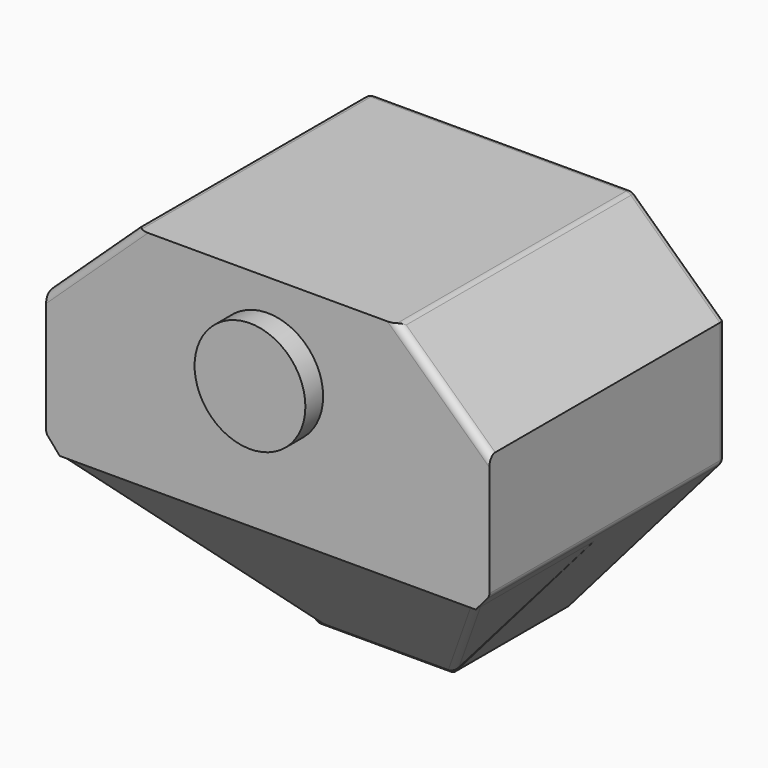
from build123d import *

# Parameters (mm, degrees)
F0_W          = 92.273324728
F0_H          = 57.6515942812
F0_W_2        = 42.1701818705
F0_H_2        = 26.3371020555
F0_H_3        = 119.797244668
F0_H_4        = 35.8085483313
F1_DEPTH      = 100
F1_DEPTH_BACK = 100
F3_DEPTH      = 100
F5_DEPTH      = 150
F5_DEPTH_BACK = 150
F7_DEPTH      = 100
F8_R          = 5
F9_T1_DEPTH   = 199.6642420397
F9_T3_DEPTH   = 100.7064549822
F9_T5_DEPTH   = 109.4378575727
F9_T7_DEPTH   = 199.9314988793
F9_T9_DEPTH   = 109.4378575727
F9_T11_DEPTH  = 200.4273166446
F9_T16_DEPTH  = 5.1
F9_T22_DEPTH  = 5.1
F9_T28_DEPTH  = 5.1
F9_T34_DEPTH  = 5.1
F9_T40_DEPTH  = 5.1
F9_T46_DEPTH  = 5.1
F9_T52_DEPTH  = 5.1
F9_T58_DEPTH  = 190.7815844726
F9_T64_DEPTH  = 191.1757464634
F10_R         = 37.5
F11_DEPTH     = 15
F12_W         = 12.8494501114
F12_H         = 17.9891586304
F13_DEPTH     = 50


# Not quite as in the source:
# - a fillet or chamfer that OpenCascade refuses, or shapes differently, is made with other operations: its cross-section is extruded or revolved along the edge and cut away or added


with BuildPart() as f1:
    # F0 (on Front) → F1 (new body, two sides)
    with BuildSketch(Plane.XZ) as f1_sk:
        with Locations((0, 13.1685510278)):
            Rectangle(F0_W, F0_H)
        with Locations((-67.2217532992, 13.1685510278)):
            Rectangle(F0_W_2, F0_H)
        Polygon((-150, 41.9943481684), (-150, -41.9943481684), (-46.136662364, -41.9943481684), (-46.136662364, -15.6572461128), (-88.3068442345, -15.6572461128), (-88.3068442345, 41.9943481684), align=None)
        with Locations((0, -28.8257971406)):
            Rectangle(F0_W, F0_H_2)
        Polygon((46.136662364, -15.6572461128), (46.136662364, -41.9943481684), (150, -41.9943481684), (150, 41.9943481684), (88.3068442345, 41.9943481684), (88.3068442345, -15.6572461128), align=None)
        with Locations((67.2217532992, 13.1685510278)):
            Rectangle(F0_W_2, F0_H)
        Polygon((-46.136662364, -41.9943481684), (-150, -41.9943481684), (-46.136662364, -161.7915928364), align=None)
        with Locations((0, -101.8929705024)):
            Rectangle(F0_W, F0_H_3)
        Polygon((150, -41.9943481684), (46.136662364, -41.9943481684), (46.136662364, -161.7915928364), align=None)
        Polygon((-88.3068442345, 99.6459424496), (-88.3068442345, 41.9943481684), (-46.136662364, 41.9943481684), (-46.136662364, 77.8028964996), (46.136662364, 77.8028964996), (46.136662364, 41.9943481684), (88.3068442345, 41.9943481684), (88.3068442345, 99.6459424496), align=None)
        with Locations((0, 59.898622334)):
            Rectangle(F0_W, F0_H_4)
        Polygon((-88.3068442345, 99.6459424496), (-150, 41.9943481684), (-88.3068442345, 41.9943481684), align=None)
        Polygon((150, 41.9943481684), (88.3068442345, 99.6459424496), (88.3068442345, 41.9943481684), align=None)
    extrude(amount=F1_DEPTH)
    extrude(f1_sk.sketch, amount=-F1_DEPTH_BACK)

    # F2 (on face) → F3 (cut)
    with BuildSketch(Plane.XZ.offset(100)):
        Polygon((140.7758174747, -52.633633175), (-140.7758174747, -52.633633175), (-46.136662364, -161.7915928364), (46.136662364, -161.7915928364), align=None)
    extrude(amount=-F3_DEPTH, mode=Mode.SUBTRACT)

    # F4 (on Right) → F5 (join, two sides)
    with BuildSketch(Plane.YZ) as f5_sk:
        Polygon((-99.6227860451, -52.5650829077), (0, -161.33877635), (0, -52.5650829077), align=None)
    extrude(amount=F5_DEPTH)
    extrude(f5_sk.sketch, amount=-F5_DEPTH_BACK)

    # F6 (on face) → F7 (cut)
    with BuildSketch(Plane.XZ.offset(100)):
        Polygon((-140.7758174747, -52.633633175), (-150, -41.9943481684), (-150.5579352379, -161.6920530796), (-44.7144806385, -161.6920530796), (-140.6417366282, -52.633633175), align=None)
        Polygon((140.7758174747, -52.633633175), (140.7202282019, -52.633633175), (45.5975532532, -161.6920530796), (150, -161.6920530796), (150, -41.9943481684), align=None)
    extrude(amount=-F7_DEPTH, mode=Mode.SUBTRACT)

    # F8
    f8_edges = [f1.edges().sort_by_distance(p)[0] for p in [
        (0, 100, 99.645942),
        (119.153422, 100, 70.820145),
        (-150, 100, 0),
        (-98.068331, 100, -101.892971),
        (0, 100, -161.791593),
        (98.068331, 100, -101.892971),
        (150, 100, 0),
        (-119.153422, 100, 70.820145),
    ]]
    fillet(f8_edges, radius=F8_R)

    # F9: fillet of radius 5 on 11 edges, made by hand

    # F9_s2 → F9_t1 (cut)
    with BuildSketch(Plane.XZ.offset(-95)):
        with BuildLine():
            ThreePointArc((148.7778357345, -43.4040073885), (149.6845052392, -41.8766246542), (150, -40.1286513525))
            Line((150, -40.1286513525), (150, -41.9943481684))
            Line((150, -41.9943481684), (148.7778357345, -43.4040073885))
        make_face()
        with BuildLine():
            ThreePointArc((-150, -40.1286513525), (-149.6845052392, -41.8766246542), (-148.7778357345, -43.4040073885))
            Line((-148.7778357345, -43.4040073885), (-150, -41.9943481684))
            Line((-150, -41.9943481684), (-150, -40.1286513525))
        make_face()
    extrude(amount=F9_T1_DEPTH, mode=Mode.SUBTRACT)

    # F9_s4 → F9_t3 (cut)
    with BuildSketch(Plane.XZ.offset(-95)):
        with BuildLine():
            ThreePointArc((47.6319161056, -160.0669488724), (45.9305220173, -161.3400420326), (43.8540803711, -161.7915928364))
            Line((43.8540803711, -161.7915928364), (46.136662364, -161.7915928364))
            Line((46.136662364, -161.7915928364), (47.6319161056, -160.0669488724))
        make_face()
        with BuildLine():
            ThreePointArc((-47.6319161056, -160.0669488724), (-45.9305220173, -161.3400420326), (-43.8540803711, -161.7915928364))
            Line((-43.8540803711, -161.7915928364), (-46.136662364, -161.7915928364))
            Line((-46.136662364, -161.7915928364), (-47.6319161056, -160.0669488724))
        make_face()
    extrude(amount=F9_T3_DEPTH, mode=Mode.SUBTRACT)

    # F9_s6 → F9_t5 (cut)
    with BuildSketch(Plane(origin=(68.2577235686, 0, -63.786112688), x_dir=(0, 1, 0), z_dir=(-0.7306338358, 0, 0.6827695057))):
        with BuildLine():
            ThreePointArc((-100, -128.0979175463), (-98.5355339059, -131.6334514522), (-95, -133.0979175463))
            Line((-95, -133.0979175463), (-100, -133.0979175463))
            Line((-100, -133.0979175463), (-100, -128.0979175463))
        make_face()
    extrude(amount=F9_T5_DEPTH, mode=Mode.SUBTRACT)

    # F9_s8 → F9_t7 (cut)
    with BuildSketch(Plane.XZ.offset(-95)):
        with BuildLine():
            ThreePointArc((86.3342446827, 99.6459424496), (88.1692043696, 99.2970630616), (89.7480922115, 98.2991116286))
            Line((89.7480922115, 98.2991116286), (88.3068442345, 99.6459424496))
            Line((88.3068442345, 99.6459424496), (86.3342446827, 99.6459424496))
        make_face()
        with BuildLine():
            ThreePointArc((-89.7480922115, 98.2991116286), (-88.1692043696, 99.2970630616), (-86.3342446827, 99.6459424496))
            Line((-86.3342446827, 99.6459424496), (-88.3068442345, 99.6459424496))
            Line((-88.3068442345, 99.6459424496), (-89.7480922115, 98.2991116286))
        make_face()
    extrude(amount=F9_T7_DEPTH, mode=Mode.SUBTRACT)

    # F9_s10 → F9_t9 (cut)
    with BuildSketch(Plane(origin=(11.701278092, 0, 10.9347192369), x_dir=(0, 1, 0), z_dir=(-0.7306338358, 0, -0.6827695057))):
        with BuildLine():
            ThreePointArc((-95, -133.0979175463), (-98.5355339059, -131.6334514522), (-100, -128.0979175463))
            Line((-100, -128.0979175463), (-100, -133.0979175463))
            Line((-100, -133.0979175463), (-95, -133.0979175463))
        make_face()
    extrude(amount=F9_T9_DEPTH, mode=Mode.SUBTRACT)

    # F9_s12 → F9_t11 (cut)
    with BuildSketch(Plane.XZ.offset(-95)):
        with BuildLine():
            ThreePointArc((-150, 39.8234215105), (-149.5863513627, 41.8147479976), (-148.4138475287, 43.4765906896))
            Line((-148.4138475287, 43.4765906896), (-150, 41.9943481684))
            Line((-150, 41.9943481684), (-150, 39.8234215105))
        make_face()
    extrude(amount=F9_T11_DEPTH, mode=Mode.SUBTRACT)


with BuildPart() as f9_tool14:
    # F9_s15 → F9_t16 (new body)
    with BuildSketch(Plane.XZ.offset(-95)):
        Polygon((-43.8540803711, -156.7915928364), (-47.7074728203, -160.1324559932), (-46.1823140039, -161.8915928364), (-43.8540803711, -161.8915928364), align=None)
    extrude(amount=-F9_T16_DEPTH)

    # F9_s17 → F9_t18 (revolve, cut)
    with BuildSketch(Plane(origin=(-43.8540803711, 95, -156.7915928364), x_dir=(0.4152883292, 0, 0.9096898392), z_dir=(-0.9096898392, 0, 0.4152883292))):
        with BuildLine():
            ThreePointArc((0, -5), (5, 0), (0, 5))
            Line((0, 5), (0, -5))
        make_face()
    revolve(axis=Axis((-43.8540803711, 95, -156.7915928364), (0, 1, 0)), mode=Mode.SUBTRACT)


with BuildPart() as f1_1:
    add(f1.part)

    # F9_t13: cut F9_tool14
    add(f9_tool14.part, mode=Mode.SUBTRACT)


with BuildPart() as f9_tool20:
    # F9_s21 → F9_t22 (new body)
    with BuildSketch(Plane.XZ.offset(-95)):
        Polygon((-145, -40.1286513525), (-150.1, -40.1286513525), (-150.1, -42.0316621047), (-148.8533924492, -43.4695145093), align=None)
    extrude(amount=-F9_T22_DEPTH)

    # F9_s23 → F9_t24 (revolve, cut)
    with BuildSketch(Plane(origin=(-145, 95, -40.1286513525), x_dir=(0.9369010478, 0, 0.3495946604), z_dir=(-0.3495946604, 0, 0.9369010478))):
        with BuildLine():
            ThreePointArc((0, -5), (5, 0), (0, 5))
            Line((0, 5), (0, -5))
        make_face()
    revolve(axis=Axis((-145, 95, -40.1286513525), (0, 1, 0)), mode=Mode.SUBTRACT)


with BuildPart() as f1_2:
    add(f1_1.part)

    # F9_t19: cut F9_tool20
    add(f9_tool20.part, mode=Mode.SUBTRACT)


with BuildPart() as f9_tool26:
    # F9_s27 → F9_t28 (new body)
    with BuildSketch(Plane.XZ.offset(-95)):
        Polygon((-145, 39.8234215105), (-150.1, 39.8234215105), (-150.1, 42.0377667015), (-148.4821244793, 43.5496540731), align=None)
    extrude(amount=-F9_T28_DEPTH)

    # F9_s29 → F9_t30 (revolve, cut)
    with BuildSketch(Plane(origin=(-145, 95, 39.8234215105), x_dir=(0.9172702725, 0, -0.3982652974), z_dir=(0.3982652974, 0, 0.9172702725))):
        with BuildLine():
            ThreePointArc((0, -5), (5, 0), (0, 5))
            Line((0, 5), (0, -5))
        make_face()
    revolve(axis=Axis((-145, 95, 39.8234215105), (0, 1, 0)), mode=Mode.SUBTRACT)


with BuildPart() as f1_3:
    add(f1_2.part)

    # F9_t25: cut F9_tool26
    add(f9_tool26.part, mode=Mode.SUBTRACT)


with BuildPart() as f9_tool32:
    # F9_s33 → F9_t34 (new body)
    with BuildSketch(Plane.XZ.offset(-95)):
        Polygon((-86.3342446827, 94.6459424496), (-89.816369162, 98.3721750122), (-88.3462962255, 99.7459424496), (-86.3342446827, 99.7459424496), align=None)
    extrude(amount=-F9_T34_DEPTH)

    # F9_s35 → F9_t36 (revolve, cut)
    with BuildSketch(Plane(origin=(-86.3342446827, 95, 94.6459424496), x_dir=(0.3669919374, 0, -0.9302241224), z_dir=(0.9302241224, 0, 0.3669919374))):
        with BuildLine():
            ThreePointArc((0, -5), (5, 0), (0, 5))
            Line((0, 5), (0, -5))
        make_face()
    revolve(axis=Axis((-86.3342446827, 95, 94.6459424496), (0, 1, 0)), mode=Mode.SUBTRACT)


with BuildPart() as f1_4:
    add(f1_3.part)

    # F9_t31: cut F9_tool32
    add(f9_tool32.part, mode=Mode.SUBTRACT)


with BuildPart() as f9_tool38:
    # F9_s39 → F9_t40 (new body)
    with BuildSketch(Plane.XZ.offset(-95)):
        Polygon((86.3342446827, 94.6459424496), (86.3342446827, 99.7459424496), (88.3462962255, 99.7459424496), (89.816369162, 98.3721750122), align=None)
    extrude(amount=-F9_T40_DEPTH)

    # F9_s41 → F9_t42 (revolve, cut)
    with BuildSketch(Plane(origin=(86.3342446827, 95, 94.6459424496), x_dir=(-0.3669919374, 0, -0.9302241224), z_dir=(0.9302241224, 0, -0.3669919374))):
        with BuildLine():
            ThreePointArc((0, -5), (5, 0), (0, 5))
            Line((0, 5), (0, -5))
        make_face()
    revolve(axis=Axis((86.3342446827, 95, 94.6459424496), (0, 1, 0)), mode=Mode.SUBTRACT)


with BuildPart() as f1_5:
    add(f1_4.part)

    # F9_t37: cut F9_tool38
    add(f9_tool38.part, mode=Mode.SUBTRACT)


with BuildPart() as f9_tool44:
    # F9_s45 → F9_t46 (new body)
    with BuildSketch(Plane.XZ.offset(-95)):
        Polygon((43.8540803711, -156.7915928364), (47.7074728203, -160.1324559932), (46.1823140039, -161.8915928364), (43.8540803711, -161.8915928364), align=None)
    extrude(amount=-F9_T46_DEPTH)

    # F9_s47 → F9_t48 (revolve, cut)
    with BuildSketch(Plane(origin=(43.8540803711, 95, -156.7915928364), x_dir=(-0.4152883292, 0, 0.9096898392), z_dir=(-0.9096898392, 0, -0.4152883292))):
        with BuildLine():
            ThreePointArc((0, -5), (5, 0), (0, 5))
            Line((0, 5), (0, -5))
        make_face()
    revolve(axis=Axis((43.8540803711, 95, -156.7915928364), (0, 1, 0)), mode=Mode.SUBTRACT)


with BuildPart() as f1_6:
    add(f1_5.part)

    # F9_t43: cut F9_tool44
    add(f9_tool44.part, mode=Mode.SUBTRACT)


with BuildPart() as f9_tool50:
    # F9_s51 → F9_t52 (new body)
    with BuildSketch(Plane.XZ.offset(-95)):
        Polygon((145, -40.1286513525), (148.8533924492, -43.4695145093), (150.1, -42.0316621047), (150.1, -40.1286513525), align=None)
    extrude(amount=-F9_T52_DEPTH)

    # F9_s53 → F9_t54 (revolve, cut)
    with BuildSketch(Plane(origin=(145, 95, -40.1286513525), x_dir=(-0.9369010478, 0, 0.3495946604), z_dir=(-0.3495946604, 0, -0.9369010478))):
        with BuildLine():
            ThreePointArc((0, -5), (5, 0), (0, 5))
            Line((0, 5), (0, -5))
        make_face()
    revolve(axis=Axis((145, 95, -40.1286513525), (0, 1, 0)), mode=Mode.SUBTRACT)


with BuildPart() as f1_7:
    add(f1_6.part)

    # F9_t49: cut F9_tool50
    add(f9_tool50.part, mode=Mode.SUBTRACT)


with BuildPart() as f9_tool56:
    # F9_s57 → F9_t58 (new body)
    with BuildSketch(Plane(origin=(-44.8947175454, 47.1416954329, -51.4719225484), x_dir=(0.7241543113, 0.6896379727, 0), z_dir=(0.5409695578, -0.5680450514, 0.6202231511))):
        with BuildLine():
            ThreePointArc((35.8427850372, -144.5001725374), (33.2234593548, -145.3091827818), (30.5712639561, -144.6154795512))
            Line((30.5712639561, -144.6154795512), (33.2428014748, -146.1934515657))
            Line((33.2428014748, -146.1934515657), (35.8427850372, -144.5001725374))
        make_face()
    extrude(amount=F9_T58_DEPTH)

    split(bisect_by=Plane.XY.offset(-52.633633175), keep=Keep.BOTTOM)

    split(bisect_by=Plane.XZ, keep=Keep.TOP)


with BuildPart() as f1_8:
    add(f1_7.part)

    # F9_t55: cut F9_tool56
    add(f9_tool56.part, mode=Mode.SUBTRACT)


with BuildPart() as f9_tool62:
    # F9_s63 → F9_t64 (new body)
    with BuildSketch(Plane(origin=(-58.840223556, -61.2669557127, 66.8946666059), x_dir=(-0.7212464746, 0.6926785134, 0), z_dir=(0.544194194, 0.5666382547, -0.6186871323))):
        with BuildLine():
            ThreePointArc((29.8139114642, -144.4686613021), (32.4583698037, -145.1693847909), (35.0757673211, -144.3735182485))
            Line((35.0757673211, -144.3735182485), (32.4742820088, -146.0494041555))
            Line((32.4742820088, -146.0494041555), (29.8139114642, -144.4686613021))
        make_face()
    extrude(amount=F9_T64_DEPTH)

    split(bisect_by=Plane.XY.offset(-52.633633175), keep=Keep.BOTTOM)

    split(bisect_by=Plane.XZ, keep=Keep.TOP)


with BuildPart() as f1_9:
    add(f1_8.part)

    # F9_t61: cut F9_tool62
    add(f9_tool62.part, mode=Mode.SUBTRACT)

    # F10 (on face) → F11 (join)
    with BuildSketch(Plane.XZ.offset(100)):
        with Locations((0, 40.7927632332)):
            Circle(F10_R)
    extrude(amount=F11_DEPTH)

    # F12 (on face) → F13 (cut)
    with BuildSketch(Plane(origin=(0, 0, -161.7915928364), x_dir=(1, 0, 0), z_dir=(0, 0, -1))):
        with Locations((27.2407829762, -29.2492955923)):
            Rectangle(F12_W, F12_H)
    extrude(amount=-F13_DEPTH, mode=Mode.SUBTRACT)


solid = f1_9.part
